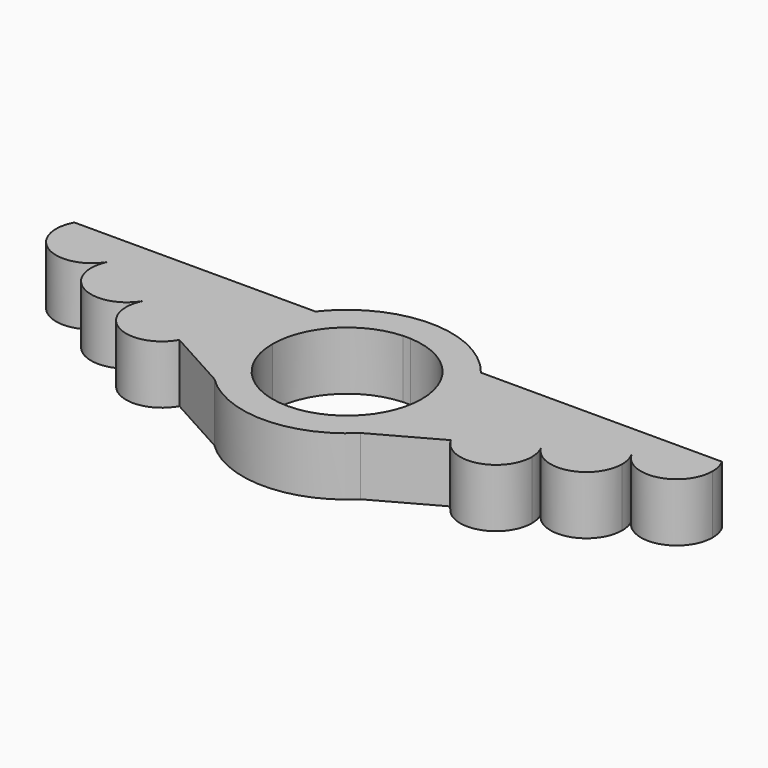
from build123d import *

# Parameters (mm, degrees)
F1_DEPTH = 24.85502


# Not quite as in the source:
# - ends of sketch curves that miss each other by under 0.0002 mm in the source are joined


with BuildPart() as f1:
    # F0 (on Top) → F1 (new body)
    with BuildSketch(Plane.XY):
        with BuildLine():
            Line((31.75, -31.7133048595), (44.45, -31.7133048595))
            ThreePointArc((44.45, -31.7133048595), (42.0664322772, -17.3530202013), (35.171359934, -4.5328350256))
            ThreePointArc((35.171359934, -4.5328350256), (33.2360090694, -2.1977123508), (31.1459274206, 0))
            Line((31.1459274206, 0), (1.526038953, 0))
            ThreePointArc((1.526038953, 0), (22.9838447258, -9.8088445461), (31.75, -31.7133048595))
        make_face()
        with BuildLine():
            Line((44.45, -40.8569961303), (44.45, -31.7133048595))
            ThreePointArc((44.45, -31.7133048595), (44.2101126583, -36.3250766164), (43.4930398768, -40.8870708405))
            ThreePointArc((43.4930398768, -40.8870708405), (43.9712837047, -40.8645166634), (44.45, -40.8569961303))
        make_face()
        with BuildLine():
            ThreePointArc((43.4930398768, -40.8870708405), (44.2101126583, -36.3250766164), (44.45, -31.7133048595))
            Line((44.45, -31.7133048595), (31.75, -31.7133048595))
            ThreePointArc((31.75, -31.7133048595), (22.4506403027, -54.1639451622), (0, -63.4633048595))
            Line((0, -63.4633048595), (31.1085197333, -63.4633048595))
            ThreePointArc((31.1085197333, -63.4633048595), (31.0883782789, -48.7672850184), (43.4930398768, -40.8870708405))
        make_face()
        with BuildLine():
            ThreePointArc((35.171359934, -4.5328350256), (42.0664322772, -17.3530202013), (44.45, -31.7133048595))
            Line((44.45, -31.7133048595), (44.45, -4.5328350256))
            Line((44.45, -4.5328350256), (35.171359934, -4.5328350256))
        make_face()
        with BuildLine():
            Line((44.45, -4.5328350256), (44.45, -31.7133048595))
            Line((44.45, -31.7133048595), (44.45, -40.8569961303))
            ThreePointArc((44.45, -40.8569961303), (52.1958071052, -42.9722076639), (57.7914802832, -48.730687431))
            ThreePointArc((57.7914802832, -48.730687431), (63.7666518684, -28.0228983697), (84.4744408875, -33.9980701011))
            ThreePointArc((84.4744408875, -33.9980701011), (90.4496122897, -13.290280973), (111.1574013682, -19.2654525473))
            ThreePointArc((111.1574013682, -19.2654525473), (109.2588815999, -11.8991437909), (111.1574013333, -4.5328350256))
            Line((111.1574013333, -4.5328350256), (44.45, -4.5328350256))
        make_face()
        with BuildLine():
            ThreePointArc((44.45, -40.8569961303), (43.9712837047, -40.8645166634), (43.4930398768, -40.8870708405))
            ThreePointArc((43.4930398768, -40.8870708405), (38.9713966864, -53.0916289358), (31.1085197333, -63.4633048595))
            Line((31.1085197333, -63.4633048595), (44.45, -56.0969961303))
            Line((44.45, -56.0969961303), (44.45, -40.8569961303))
        make_face()
        with BuildLine():
            ThreePointArc((31.1085197333, -63.4633048595), (38.9713966864, -53.0916289358), (43.4930398768, -40.8870708405))
            ThreePointArc((43.4930398768, -40.8870708405), (31.0883782789, -48.7672850184), (31.1085197333, -63.4633048595))
        make_face()
        with BuildLine():
            ThreePointArc((57.7914802832, -48.730687431), (52.1958071052, -42.9722076639), (44.45, -40.8569961303))
            Line((44.45, -40.8569961303), (44.45, -56.0969961303))
            Line((44.45, -56.0969961303), (57.7914802667, -48.7306874011))
        make_face()
        with BuildLine():
            Line((1.526038953, 0), (31.1459274206, 0))
            ThreePointArc((31.1459274206, 0), (0, 12.7366951405), (-31.1459274206, 0))
            Line((-31.1459274206, 0), (-1.526038953, 0))
            ThreePointArc((-1.526038953, 0), (0, 0.0366951405), (1.526038953, 0))
        make_face()
        with BuildLine():
            ThreePointArc((-31.1085197333, -63.4633048595), (0, -76.1633048595), (31.1085197333, -63.4633048595))
            Line((31.1085197333, -63.4633048595), (0, -63.4633048595))
            Line((0, -63.4633048595), (-31.1085197333, -63.4633048595))
        make_face()
        with BuildLine():
            Line((-31.1085197333, -63.4633048595), (0, -63.4633048595))
            ThreePointArc((0, -63.4633048595), (-22.4506403027, -54.1639451622), (-31.75, -31.7133048595))
            Line((-31.75, -31.7133048595), (-44.45, -31.7133048595))
            ThreePointArc((-44.45, -31.7133048595), (-44.2101126583, -36.3250766164), (-43.4930398768, -40.8870708405))
            ThreePointArc((-43.4930398768, -40.8870708405), (-33.340506936, -45.6645101437), (-29.21, -56.0969961303))
            ThreePointArc((-29.21, -56.0969961303), (-29.6922603481, -59.9005103432), (-31.1085197333, -63.4633048595))
        make_face()
        with BuildLine():
            Line((137.8403618666, -4.5328350256), (111.1574013333, -4.5328350256))
            ThreePointArc((111.1574013333, -4.5328350256), (109.2588815999, -11.8991437909), (111.1574013682, -19.2654525473))
            Line((111.1574013333, -19.2654524841), (137.8403618666, -4.5328350256))
        make_face()
        with BuildLine():
            ThreePointArc((84.4744408875, -33.9980701011), (63.7666518684, -28.0228983697), (57.7914802832, -48.730687431))
            Line((57.7914802832, -48.730687431), (84.4744408875, -33.9980701011))
        make_face()
        with BuildLine():
            Line((84.4744408, -33.9980699426), (57.7914802667, -48.7306874011))
            ThreePointArc((57.7914802667, -48.7306874011), (74.9364747628, -56.1221183194), (86.3729605333, -41.3643786718))
            ThreePointArc((86.3729605333, -41.3643786718), (85.8907002078, -37.5608645466), (84.4744408, -33.9980699426))
        make_face()
        with BuildLine():
            Line((-1.526038953, 0), (-31.1459274206, 0))
            ThreePointArc((-31.1459274206, 0), (-33.2360090694, -2.1977123508), (-35.171359934, -4.5328350256))
            ThreePointArc((-35.171359934, -4.5328350256), (-42.0664322772, -17.3530202013), (-44.45, -31.7133048595))
            Line((-44.45, -31.7133048595), (-31.75, -31.7133048595))
            ThreePointArc((-31.75, -31.7133048595), (-22.9838447258, -9.8088445461), (-1.526038953, 0))
        make_face()
        with BuildLine():
            Line((-44.45, -56.0969961303), (-31.1085197333, -63.4633048595))
            ThreePointArc((-31.1085197333, -63.4633048595), (-38.9713966864, -53.0916289358), (-43.4930398768, -40.8870708405))
            ThreePointArc((-43.4930398768, -40.8870708405), (-43.9712837047, -40.8645166634), (-44.45, -40.8569961303))
            Line((-44.45, -40.8569961303), (-44.45, -56.0969961303))
        make_face()
        with BuildLine():
            ThreePointArc((-43.4930398768, -40.8870708405), (-38.9713966864, -53.0916289358), (-31.1085197333, -63.4633048595))
            ThreePointArc((-31.1085197333, -63.4633048595), (-29.6922603481, -59.9005103432), (-29.21, -56.0969961303))
            ThreePointArc((-29.21, -56.0969961303), (-33.340506936, -45.6645101437), (-43.4930398768, -40.8870708405))
        make_face()
        with BuildLine():
            ThreePointArc((113.0559210666, -26.6317612133), (112.5736607275, -22.8282470353), (111.1574013682, -19.2654525473))
            Line((111.1574013682, -19.2654525473), (84.4744408, -33.9980699426))
            ThreePointArc((84.4744408, -33.9980699426), (101.6194353672, -41.3895008426), (113.0559210666, -26.6317612133))
        make_face()
        with BuildLine():
            Line((84.4744408, -33.9980699426), (111.1574013333, -19.2654524841))
            ThreePointArc((111.1574013333, -19.2654524841), (90.4496122897, -13.290280973), (84.4744408, -33.9980699426))
        make_face()
        with BuildLine():
            Line((137.8403618666, -4.5328350256), (111.1574013333, -19.2654524841))
            ThreePointArc((111.1574013682, -19.2654525473), (128.3023958478, -26.6568833977), (139.7388815999, -11.8991437549))
            ThreePointArc((139.7388815999, -11.8991437549), (139.2566212518, -8.0956295419), (137.8403618666, -4.5328350256))
        make_face()
        with BuildLine():
            ThreePointArc((-44.45, -31.7133048595), (-42.0664322772, -17.3530202013), (-35.171359934, -4.5328350256))
            Line((-35.171359934, -4.5328350256), (-111.1574013333, -4.5328350256))
            ThreePointArc((-111.1574013333, -4.5328350256), (-109.7411419481, -8.0956295419), (-109.2588815999, -11.8991437548))
            ThreePointArc((-109.2588815999, -11.8991437548), (-109.7411419274, -15.7026578875), (-111.1574012531, -19.265452339))
            ThreePointArc((-111.1574012531, -19.265452339), (-94.0124067734, -11.8740215822), (-82.5759210666, -26.6317612133))
            ThreePointArc((-82.5759210666, -26.6317612133), (-83.058181437, -30.4352755127), (-84.4744408863, -33.9980700989))
            ThreePointArc((-84.4744408863, -33.9980700989), (-67.3294464068, -26.6066389977), (-55.8929605333, -41.3643786718))
            ThreePointArc((-55.8929605333, -41.3643786718), (-56.3752208889, -45.1678929135), (-57.7914802953, -48.730687453))
            ThreePointArc((-57.7914802953, -48.730687453), (-52.1958071161, -42.9722076703), (-44.45, -40.8569961303))
            Line((-44.45, -40.8569961303), (-44.45, -31.7133048595))
        make_face()
        with BuildLine():
            ThreePointArc((-44.45, -40.8569961303), (-43.9712837047, -40.8645166634), (-43.4930398768, -40.8870708405))
            ThreePointArc((-43.4930398768, -40.8870708405), (-44.2101126583, -36.3250766164), (-44.45, -31.7133048595))
            Line((-44.45, -31.7133048595), (-44.45, -40.8569961303))
        make_face()
        with BuildLine():
            Line((-57.7914802667, -48.7306874011), (-44.45, -56.0969961303))
            Line((-44.45, -56.0969961303), (-44.45, -40.8569961303))
            ThreePointArc((-44.45, -40.8569961303), (-52.1958071161, -42.9722076703), (-57.7914802953, -48.730687453))
        make_face()
        with BuildLine():
            ThreePointArc((-84.4744408863, -33.9980700989), (-78.4992692104, -54.7058589673), (-57.7914802953, -48.730687453))
            Line((-57.7914802953, -48.730687453), (-84.4744408863, -33.9980700989))
        make_face()
        with BuildLine():
            Line((-84.4744408, -33.9980699426), (-57.7914802667, -48.7306874011))
            ThreePointArc((-57.7914802667, -48.7306874011), (-56.3752208889, -45.1678929135), (-55.8929605333, -41.3643786718))
            ThreePointArc((-55.8929605333, -41.3643786718), (-67.3294464068, -26.6066389977), (-84.4744408, -33.9980699426))
        make_face()
        with BuildLine():
            ThreePointArc((-109.2588815999, -11.8991437548), (-109.7411419481, -8.0956295419), (-111.1574013333, -4.5328350256))
            Line((-111.1574013333, -4.5328350256), (-137.8403618666, -4.5328350256))
            Line((-137.8403618666, -4.5328350256), (-111.1574013333, -19.2654524841))
            ThreePointArc((-111.1574013333, -19.2654524841), (-109.7411419274, -15.7026578875), (-109.2588815999, -11.8991437548))
        make_face()
        with BuildLine():
            ThreePointArc((-111.1574012531, -19.265452339), (-105.1822299466, -39.9732413968), (-84.4744408863, -33.9980700989))
            Line((-84.4744408863, -33.9980700989), (-111.1574012531, -19.265452339))
        make_face()
        with BuildLine():
            Line((-111.1574013333, -19.2654524841), (-84.4744408, -33.9980699426))
            ThreePointArc((-84.4744408, -33.9980699426), (-83.058181437, -30.4352755127), (-82.5759210666, -26.6317612133))
            ThreePointArc((-82.5759210666, -26.6317612133), (-94.0124067734, -11.8740215822), (-111.1574013333, -19.2654524841))
        make_face()
        with BuildLine():
            Line((-111.1574013333, -19.2654524841), (-137.8403618666, -4.5328350256))
            ThreePointArc((-137.8403618666, -4.5328350256), (-131.8651902566, -25.2406240616), (-111.1574013333, -19.2654524841))
        make_face()
    extrude(amount=F1_DEPTH)


solid = f1.part
